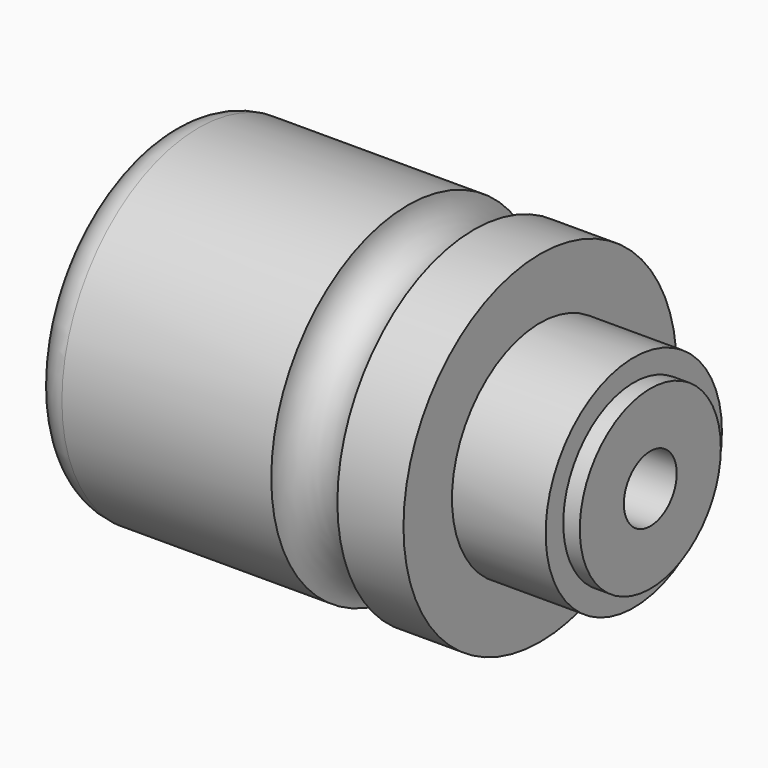
from build123d import *

# Parameters (mm, degrees)
F2_R = 5.99999


# Not quite as in the source:
# - a fillet or chamfer is up to 0.001 mm smaller than in the source, because OpenCascade refuses the exact size


with BuildPart() as f1:
    # F0 (on Top) → F1 (revolve)
    with BuildSketch(Plane.XY):
        with BuildLine():
            Line((-32.2816833258, 6), (25.7183166742, 6))
            Line((25.7183166742, 6), (25.7183166742, 16))
            Line((25.7183166742, 16), (22.7183166742, 16))
            Line((22.7183166742, 16), (22.7183166742, 20))
            Line((22.7183166742, 20), (5.7183166742, 20))
            Line((5.7183166742, 20), (5.7183166742, 31))
            Line((5.7183166742, 31), (-6.2816833258, 31))
            ThreePointArc((-6.2816833258, 31), (-12.2816833258, 25.0169717373), (-18.2816833258, 31))
            Line((-18.2816833258, 31), (-62.2816833258, 31))
            Line((-62.2816833258, 31), (-62.2816833258, 25))
            Line((-62.2816833258, 25), (-60.7816833258, 25))
            Line((-60.7816833258, 25), (-60.7816833258, 16))
            Line((-60.7816833258, 16), (-48.7816833258, 16))
            Line((-48.7816833258, 16), (-48.7816833258, 13.4885394946))
            Line((-48.7816833258, 13.4885394946), (-45.7816833258, 13.4885394946))
            Line((-45.7816833258, 13.4885394946), (-45.7816833258, 20.5))
            Line((-45.7816833258, 20.5), (-40.2816833258, 20.5))
            Line((-40.2816833258, 20.5), (-40.2816833258, 16))
            Line((-40.2816833258, 16), (-32.2816833258, 16))
            Line((-32.2816833258, 16), (-32.2816833258, 6))
        make_face()
    revolve(axis=Axis((-40.0854273438, 0, 0), (1, 0, 0)))

    # F2 (radius 6 in the source; OpenCascade refuses exactly that, so slightly less here)
    f2_edges = [f1.edges().sort_by_distance(p)[0] for p in [
        (-62.281683, -31, 0),
    ]]
    fillet(f2_edges, radius=F2_R)


solid = f1.part
